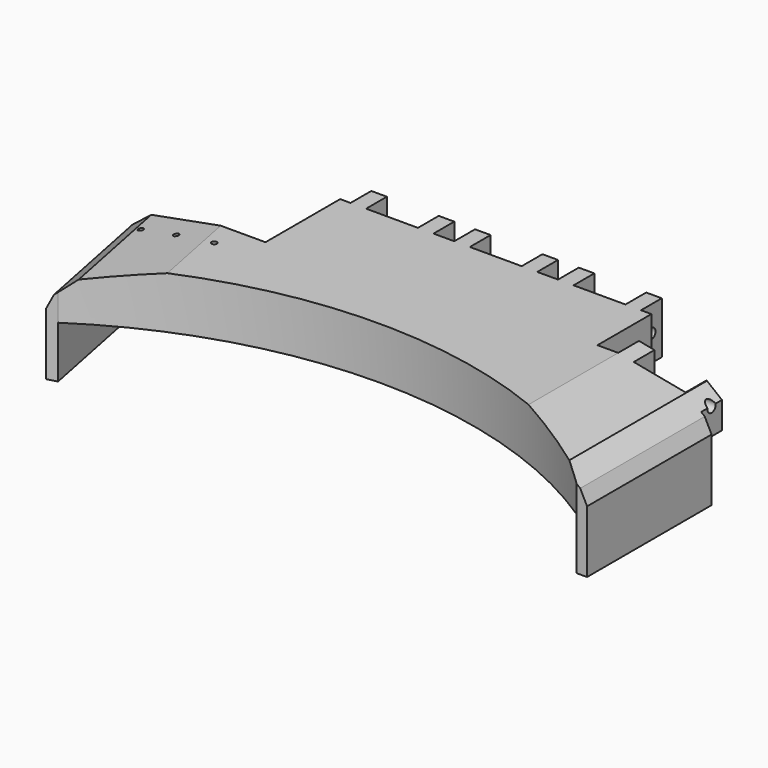
from build123d import *

# Parameters (mm, degrees)
F1_DEPTH     = 12.7
F0_W         = 2.54
F0_H         = 38.1
F2_DEPTH     = 12.7
F4_D         = 1.27
F5_W         = 3.81
F5_H         = 12.7
F6_DEPTH     = 6.35
F8_D         = 2.54
F9_W         = 3.81
F9_H         = 12.7
F10_DEPTH    = 6.35
F12_D        = 2.54
F12_DEPTH    = 22.86
F12_TIP      = 0.7630929862
F13_T1_DEPTH = 90.7253227153
F13_T3_DEPTH = 85.6453227153
F14_T1_DEPTH = 70.3362845074
F14_T3_DEPTH = 82.312532111
F15_T1_DEPTH = 94.0409858467
F15_T3_DEPTH = 99.4843801619


# Not quite as in the source:
# - a fillet or chamfer that OpenCascade refuses, or shapes differently, is made with other operations: its cross-section is extruded or revolved along the edge and cut away or added


with BuildPart() as f1:
    # F0 (on Top) → F1 (new body)
    with BuildSketch(Plane.XY):
        with BuildLine():
            ThreePointArc((-63.5, 0), (0, 19.05), (63.5, 0))
            Line((63.5, 0), (63.5, 38.1))
            Line((63.5, 38.1), (38.1, 38.1))
            Line((38.1, 38.1), (38.1, 54.61))
            Line((38.1, 54.61), (-38.1, 54.61))
            Line((-38.1, 54.61), (-38.1, 31.75))
            Line((-38.1, 31.75), (-69.85, 31.75))
            Line((-69.85, 31.75), (-63.5, 0))
        make_face()
    extrude(amount=F1_DEPTH)

    # F0 (on Top) → F2 (join, symmetric)
    with BuildSketch(Plane.XY):
        Polygon((-65.9142452177, -0.6287739113), (-63.5, 0), (-69.85, 31.75), (-72.39, 31.75), align=None)
        with Locations((64.77, 19.05)):
            Rectangle(F0_W, F0_H)
    extrude(amount=F2_DEPTH, both=True)

    # F4 (through all)
    with Locations(Plane.XY.offset(12.7)):
        with Locations((-45.604262501, 25.4304688424), (-54.9195222557, 25.4304688424), (-63.5848790407, 25.4304688424)):
            Hole(F4_D / 2)

    # F5 (on face) → F6 (join)
    with BuildSketch(Plane(origin=(0, 54.61, 0), x_dir=(-1, 0, 0), z_dir=(0, 1, 0))):
        with Locations((-33.655, 6.35)):
            Rectangle(F5_W, F5_H)
        with Locations((-17.145, 6.35)):
            Rectangle(F5_W, F5_H)
        with Locations((-8.255, 6.35)):
            Rectangle(F5_W, F5_H)
        with Locations((8.255, 6.35)):
            Rectangle(F5_W, F5_H)
        with Locations((17.145, 6.35)):
            Rectangle(F5_W, F5_H)
        with Locations((33.655, 6.35)):
            Rectangle(F5_W, F5_H)
    extrude(amount=F6_DEPTH)

    # F8 (through all)
    with Locations(Plane.YZ.offset(35.56)):
        with Locations((57.785, 6.35)):
            Hole(F8_D / 2)

    # F9 (on face) → F10 (join)
    with BuildSketch(Plane(origin=(0, 38.1, 0), x_dir=(-1, 0, 0), z_dir=(0, 1, 0))):
        with Locations((-45.085, 6.35)):
            Rectangle(F9_W, F9_H)
        with Locations((-61.595, 6.35)):
            Rectangle(F9_W, F9_H)
    extrude(amount=F10_DEPTH)

    # F12
    with Locations(Plane.YZ.offset(63.5)):
        with Locations((41.275, 6.35)):
            Hole(F12_D / 2, depth=F12_DEPTH)
            with Locations((0, 0, -(F12_DEPTH + F12_TIP / 2))):  # 118° drill point
                Cone(0, F12_D / 2, F12_TIP, mode=Mode.SUBTRACT)

    # F13: chamfer of 5.08 x 10.16 on 2 edges, made by hand

    # F13_s2 → F13_t1 (cut)
    with BuildSketch(Plane.XZ.offset(-64.4126613577)):
        Polygon((60.96, 12.7), (66.04, 2.54), (66.04, 12.7), align=None)
    extrude(amount=F13_T1_DEPTH, mode=Mode.SUBTRACT)

    # F13_s4 → F13_t3 (cut)
    with BuildSketch(Plane(origin=(-14.0503374507, 70.2516872533, 0), x_dir=(0, 0, 1), z_dir=(0.1961161351, -0.9805806757, 0))):
        Polygon((12.7, 59.6775478226), (2.54, 64.7575478226), (12.7, 64.7575478226), align=None)
    extrude(amount=F13_T3_DEPTH, mode=Mode.SUBTRACT)

    # F14: chamfer of 5.08 x 7.62 on 2 edges, made by hand

    # F14_s2 → F14_t1 (cut)
    with BuildSketch(Plane(origin=(-12.5630602506, 62.8153012532, 0), x_dir=(0, 0, 1), z_dir=(0.1961161351, -0.9805806757, 0))):
        Polygon((5.8844648046, 63.0853154203), (12.7, 54.5975478226), (12.7, 59.6775478226), align=None)
    extrude(amount=F14_T1_DEPTH, mode=Mode.SUBTRACT)

    # F14_s4 → F14_t3 (cut)
    with BuildSketch(Plane.XZ.offset(-64.1950058926)):
        Polygon((55.88, 12.7), (64.3677675977, 5.8844648046), (60.96, 12.7), align=None)
    extrude(amount=F14_T3_DEPTH, mode=Mode.SUBTRACT)

    # F15: chamfer of 12.7 x 5.08 on 2 edges, made by hand

    # F15_s2 → F15_t1 (cut)
    with BuildSketch(Plane(origin=(-14.9629972051, 74.8149860255, 0), x_dir=(0, 0, 1), z_dir=(0.1961161351, -0.9805806757, 0))):
        Polygon((12.7, 41.8975478226), (9.5193490439, 58.5585905509), (12.7, 54.5975478226), align=None)
    extrude(amount=F15_T1_DEPTH, mode=Mode.SUBTRACT)

    # F15_s4 → F15_t3 (cut)
    with BuildSketch(Plane.XZ.offset(-71.0983312548)):
        Polygon((59.8410427283, 9.5193490439), (43.18, 12.7), (55.88, 12.7), align=None)
    extrude(amount=F15_T3_DEPTH, mode=Mode.SUBTRACT)


solid = f1.part
